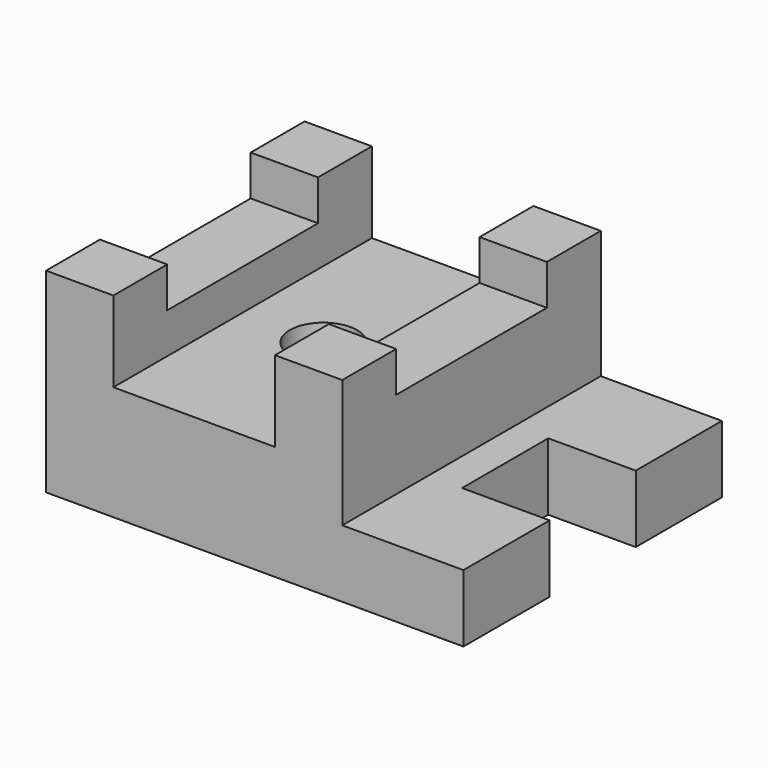
from build123d import *

# Parameters (mm, degrees)
F0_R     = 15.875
F1_DEPTH = 31.75
F0_W     = 31.75
F0_H     = 31.75
F2_DEPTH = 92.075
F0_H_2   = 88.9
F3_DEPTH = 73.025
F4_DEPTH = 53.975


with BuildPart() as f1:
    # F0 (on Top) → F1 (new body)
    with BuildSketch(Plane.XY):
        Polygon((-38.1, -44.45), (-38.1, -76.2), (38.1, -76.2), (38.1, -44.45), (38.1, 44.45), (38.1, 76.2), (-38.1, 76.2), (-38.1, 44.45), align=None)
        Circle(F0_R, mode=Mode.SUBTRACT)
    extrude(amount=F1_DEPTH)



with BuildPart() as f1b:
    # F0 (on Top) → F1, piece 2 (new body)
    with BuildSketch(Plane.XY):
        Polygon((69.85, -44.45), (69.85, -76.2), (127, -76.2), (127, -25.4), (85.725, -25.4), (85.725, 25.4), (127, 25.4), (127, 76.2), (69.85, 76.2), (69.85, 44.45), align=None)
    extrude(amount=F1_DEPTH)


with BuildPart() as f1_1:
    add(f1.part)

    add(f1b.part)  # F2 merges F1b
    # F0 (on Top) → F2 (join)
    with BuildSketch(Plane.XY):
        with Locations((-53.975, 60.325)):
            Rectangle(F0_W, F0_H)
        with Locations((53.975, 60.325)):
            Rectangle(F0_W, F0_H)
        with Locations((53.975, -60.325)):
            Rectangle(F0_W, F0_H)
        with Locations((-53.975, -60.325)):
            Rectangle(F0_W, F0_H)
    extrude(amount=F2_DEPTH)

    # F0 (on Top) → F3 (join)
    with BuildSketch(Plane.XY):
        with Locations((-53.975, 0)):
            Rectangle(F0_W, F0_H_2)
        with Locations((53.975, 0)):
            Rectangle(F0_W, F0_H_2)
    extrude(amount=F3_DEPTH)

    # F0 (on Top) → F4 (join)
    with BuildSketch(Plane.XY):
        Polygon((-38.1, -44.45), (-38.1, -76.2), (38.1, -76.2), (38.1, -44.45), (38.1, 44.45), (38.1, 76.2), (-38.1, 76.2), (-38.1, 44.45), align=None)
        Circle(F0_R, mode=Mode.SUBTRACT)
    extrude(amount=F4_DEPTH)


solid = f1_1.part
